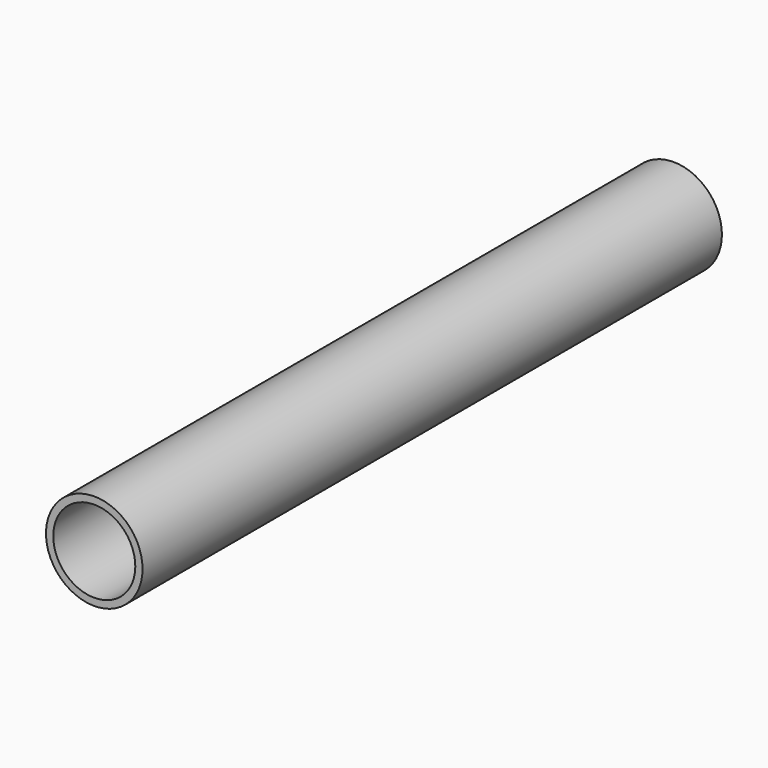
from build123d import *

# Parameters (mm, degrees)
F0_R     = 10
F0_R_2   = 8.5
F1_DEPTH = 75


# Not quite as in the source:
# - a feature names something its author has since deleted; it is built from what else it names


with BuildPart() as f1:
    # F0 (on Front) → F1 (new body, symmetric)
    with BuildSketch(Plane.XZ):
        Circle(F0_R)
        Circle(F0_R_2, mode=Mode.SUBTRACT)
    extrude(amount=F1_DEPTH, both=True)


solid = f1.part
